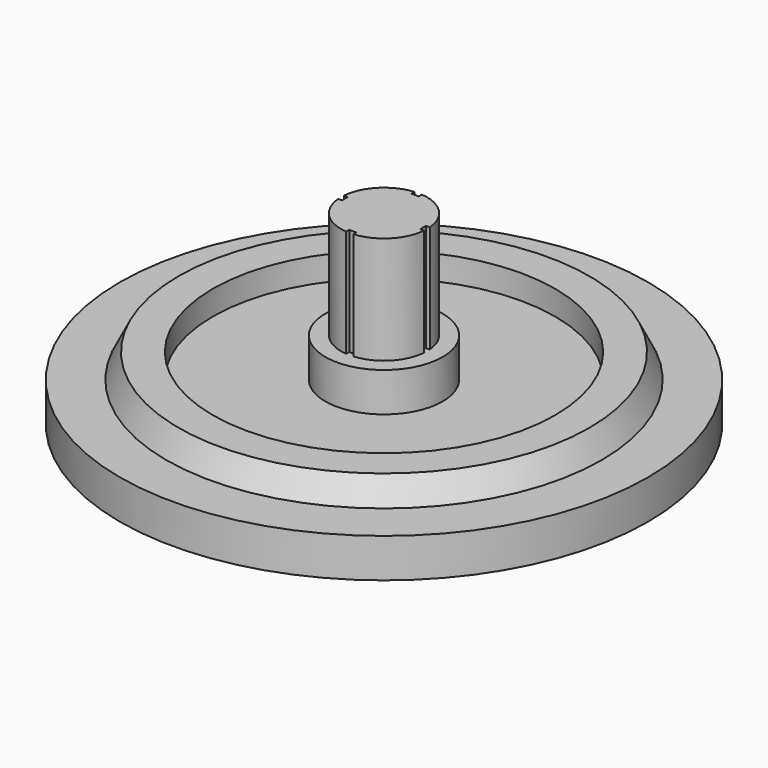
from build123d import *

# Parameters (mm, degrees)
F0_R      = 13.5
F0_R_2    = 11.25
F0_R_3    = 10.5
F0_R_4    = 8.75
F0_R_5    = 3
F0_R_6    = 2.2
F1_DEPTH  = 2
F4_DEPTH  = 1.25
F6_DEPTH  = 2
F7_DEPTH  = 2
F8_DEPTH  = 6.25
F11_DEPTH = 1.6


# Not quite as in the source:
# - a fillet or chamfer that OpenCascade refuses, or shapes differently, is made with other operations: its cross-section is extruded or revolved along the edge and cut away or added


with BuildPart() as f1:
    # F0 (on Top) → F1 (new body)
    with BuildSketch(Plane.XY):
        Circle(F0_R)
        Circle(F0_R_2, mode=Mode.SUBTRACT)
        Circle(F0_R_2)
        Circle(F0_R_3, mode=Mode.SUBTRACT)
        Circle(F0_R_3)
        Circle(F0_R_4, mode=Mode.SUBTRACT)
        Circle(F0_R_4)
        Circle(F0_R_5, mode=Mode.SUBTRACT)
        Circle(F0_R_5)
        Circle(F0_R_6, mode=Mode.SUBTRACT)
        Circle(F0_R_6)
    extrude(amount=-F1_DEPTH)

    # F0 (on Top) → F4 (join)
    with BuildSketch(Plane.XY):
        Circle(F0_R_2)
        Circle(F0_R_3, mode=Mode.SUBTRACT)
        Circle(F0_R_3)
        Circle(F0_R_4, mode=Mode.SUBTRACT)
    extrude(amount=F4_DEPTH)

    # F5: chamfer of 1.5 x 0.75 on 1 edges, made by hand


with BuildPart() as f5_tool2:
    # F5_s3 → F5_t4 (revolve)
    with BuildSketch(Plane.XZ):
        Polygon((11.25, -0.25), (10.5, 1.25), (11.25, 1.25), align=None)
    revolve(axis=Axis((0, 0, 1.25), (0, 0, 1)))

    split(bisect_by=Plane.XY, keep=Keep.TOP)


with BuildPart() as f1_1:
    add(f1.part)

    # F5_t1: cut F5_tool2
    add(f5_tool2.part, mode=Mode.SUBTRACT)

    # F0 (on Top) → F6 (join)
    with BuildSketch(Plane.XY):
        Circle(F0_R_5)
        Circle(F0_R_6, mode=Mode.SUBTRACT)
    extrude(amount=F6_DEPTH)

    # F0 (on Top) → F7 (join)
    with BuildSketch(Plane.XY):
        Circle(F0_R_6)
    extrude(amount=F7_DEPTH)

    # F3 (on offset) → F8 (join)
    with BuildSketch(Plane.XY.offset(1.25)):
        with BuildLine():
            Line((-0.1818181818, 1.9917183909), (-0.1833333333, 2.1923478029))
            ThreePointArc((-0.1833333333, 2.1923478029), (-1.5556349186, 1.5556349186), (-2.1923478029, 0.1833333333))
            Line((-2.1923478029, 0.1833333333), (-1.9917183909, 0.1818181818))
            ThreePointArc((-1.9917183909, 0.1818181818), (-2, 0), (-1.9917183909, -0.1818181818))
            Line((-1.9917183909, -0.1818181818), (-2.1923478029, -0.1833333333))
            ThreePointArc((-2.1923478029, -0.1833333333), (-1.5556349186, -1.5556349186), (-0.1833333333, -2.1923478029))
            Line((-0.1833333333, -2.1923478029), (-0.1818181818, -1.9917183909))
            ThreePointArc((-0.1818181818, -1.9917183909), (0, -2), (0.1818181818, -1.9917183909))
            Line((0.1818181818, -1.9917183909), (0.1833333333, -2.1923478029))
            ThreePointArc((0.1833333333, -2.1923478029), (1.5556349186, -1.5556349186), (2.1923478029, -0.1833333333))
            Line((2.1923478029, -0.1833333333), (1.9917183909, -0.1818181818))
            ThreePointArc((1.9917183909, -0.1818181818), (2, 0), (1.9917183909, 0.1818181818))
            Line((1.9917183909, 0.1818181818), (2.1923478029, 0.1833333333))
            ThreePointArc((2.1923478029, 0.1833333333), (1.5556349186, 1.5556349186), (0.1833333333, 2.1923478029))
            Line((0.1833333333, 2.1923478029), (0.1818181818, 1.9917183909))
            ThreePointArc((0.1818181818, 1.9917183909), (0, 2), (-0.1818181818, 1.9917183909))
        make_face()
    extrude(amount=F8_DEPTH)

    # F10 (on offset) → F11 (join)
    with BuildSketch(Plane(origin=(0, 0, -2), x_dir=(1, 0, 0), z_dir=(0, 0, -1))):
        with BuildLine():
            Line((-4.9, -7.4), (4.9, -7.4))
            ThreePointArc((4.9, -7.4), (6.667766953, -6.667766953), (7.4, -4.9))
            Line((7.4, -4.9), (7.4, 4.9))
            ThreePointArc((7.4, 4.9), (6.667766953, 6.667766953), (4.9, 7.4))
            Line((4.9, 7.4), (-4.9, 7.4))
            ThreePointArc((-4.9, 7.4), (-6.667766953, 6.667766953), (-7.4, 4.9))
            Line((-7.4, 4.9), (-7.4, -4.9))
            ThreePointArc((-7.4, -4.9), (-6.667766953, -6.667766953), (-4.9, -7.4))
        make_face()
    extrude(amount=F11_DEPTH)


solid = f1_1.part
